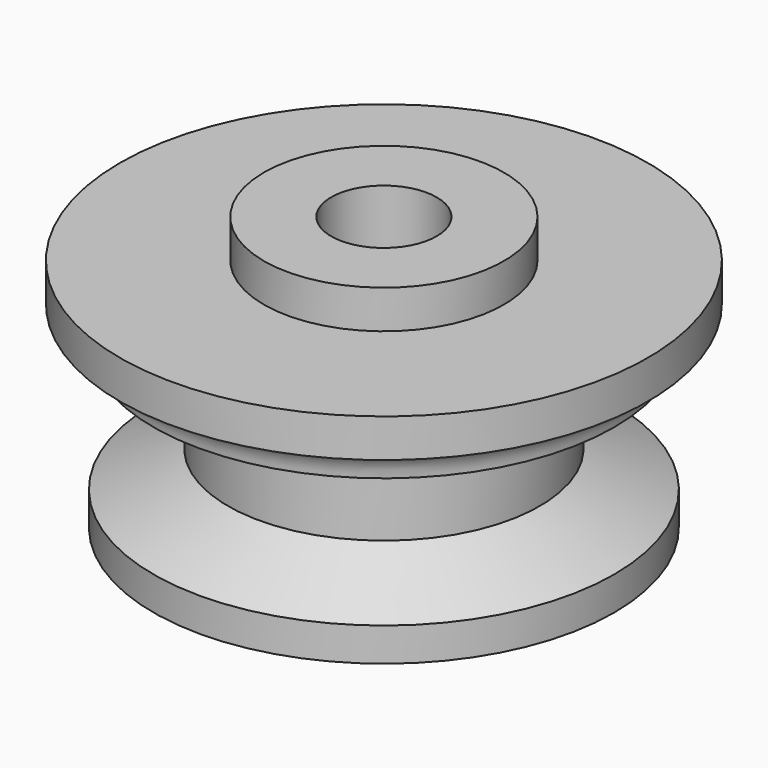
from build123d import *

# Parameters (mm, degrees)
F2_R     = 0.69999
F3_R     = 1.1
F4_DEPTH = 5.701


# Not quite as in the source:
# - a fillet or chamfer is up to 0.001 mm smaller than in the source, because OpenCascade refuses the exact size


with BuildPart() as f1:
    # F0 (on Front) → F1 (revolve)
    with BuildSketch(Plane.XZ):
        Polygon((-4.8, 0), (0, 0), (0, 5.7), (-2.5, 5.7), (-2.5, 4.9), (-5.5, 4.9), (-5.5, 4.1), (-4.8, 4.1), (-4.8, 3.4), (-3.25, 2.65), (-3.25, 1.45), (-4.8, 0.7), align=None)
    revolve(axis=Axis((0, 0, 2.85), (0, 0, -1)))

    # F2 (radius 0.7 in the source; OpenCascade refuses exactly that, so slightly less here)
    f2_edges = [f1.edges().sort_by_distance(p)[0] for p in [
        (4.8, 0, 4.1),
    ]]
    fillet(f2_edges, radius=F2_R)

    # F3 (on face) → F4 (cut, through all)
    with BuildSketch(Plane.XY.offset(5.7)):
        Circle(F3_R)
    extrude(amount=-F4_DEPTH, mode=Mode.SUBTRACT)


solid = f1.part
